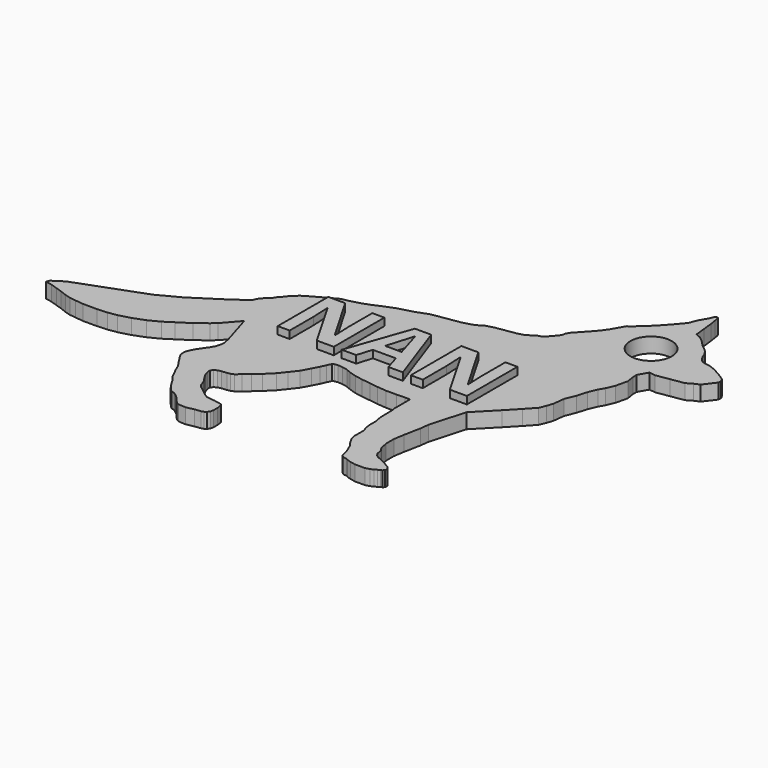
from build123d import *

# Parameters (mm, degrees)
F1_DEPTH     = 2
F2_TEXT_SIZE = 11.7813030051
F3_DEPTH     = 1
F4_R         = 2.75
F5_DEPTH     = 25


# Not quite as in the source:
# - Text() gives the source's letters only with a copy of the font that has no kerning and outlines rounded to 1/6400 em; it was checked with that copy


with BuildPart() as f1:
    # F0 (on Top) → F1 (new body)
    with BuildSketch(Plane.XY):
        Polygon((-14.7642782829, 2.6646352451), (-14.9479145184, 2.8952443972), (-15.7733522356, 3.3807961736), (-16.5259577334, 3.7813764066), (-17.0175787061, 3.969527781), (-17.4302980304, 4.218372982), (-17.7094899118, 4.7039249912), (-17.8126692772, 5.3533501923), (-18.1480534375, 5.8560813777), (-18.3847602457, 6.9182254374), (-18.3847602457, 8.2523440942), (-18.1536488235, 9.6542872488), (-17.7318826318, 11.7992078885), (-17.5875257701, 12.9829216748), (-16.272848472, 17.6499541849), (-13.6595489457, 20.3296020627), (-12.1902143583, 21.8657236546), (-11.032557115, 23.134695366), (-10.6763551012, 23.9806752652), (-10.4058505967, 24.8027704656), (-10.2194390335, 26.3313291684), (-9.6577452496, 27.7172196656), (-9.2633534223, 29.0438104421), (-8.7972544134, 30.1552768797), (-8.3670094609, 30.9082064778), (-7.900910452, 31.9838188589), (-7.5293937698, 33.5728228092), (-7.7079210069, 34.6964979394), (-7.7079210069, 35.2647826076), (-7.0022613507, 36.4996885333), (-6.1550052792, 36.3963635328), (-4.3928318448, 36.676334092), (-2.6384201724, 36.955071478), (-1.8559044693, 37.4121628702), (-1.1538827093, 37.7210527658), (0, 39.2280593514), (0, 39.6919772029), (-0.186430887, 40.0440022349), (-0.7630236214, 40.4506511986), (-1.4578301318, 40.8476829992), (-2.1245303449, 41.2286540783), (-2.869104268, 41.5249355137), (-3.3008807804, 41.639059782), (-3.839620389, 41.7309626937), (-4.1983937845, 41.8413393199), (-4.5092995279, 42.101085186), (-4.9067870714, 42.7150242031), (-5.1091215573, 43.2863943279), (-5.4541163373, 43.8192556956), (-5.84711181, 44.1954396665), (-6.3063995913, 44.533226639), (-6.6842092201, 44.9110381305), (-7.2530955076, 45.4910211265), (-7.8333392739, 45.9576323628), (-8.3694400653, 46.1709580073), (-8.5414147635, 46.2692291419), (-8.6991982535, 47.6955734193), (-8.8518235205, 49.0752879662), (-8.9826229554, 49.898557706), (-9.0659948644, 50.4233120359), (-9.1758315062, 50.5929601192), (-9.4891982153, 50.5929601192), (-9.7224124552, 50.0068780339), (-10.3918244695, 48.8354055599), (-10.823905442, 47.7495588401), (-11.8327699602, 46.5355329216), (-13.1241520867, 45.1289601624), (-14.3222687766, 44.0244451165), (-14.98264962, 43.4156558528), (-15.3725821915, 43.1631986287), (-15.7134736528, 42.5666378337), (-16.0001238116, 42.0649994351), (-16.2765689786, 41.5812197945), (-16.7349204421, 40.9167297184), (-17.23238267, 40.298666805), (-17.6576314861, 39.8354860096), (-18.3152012842, 39.119261318), (-19.0280626321, 38.3428130984), (-19.3103955608, 37.8487298621), (-19.3617039295, 37.4280056746), (-19.9972675541, 36.6383611881), (-20.6916112409, 35.8820823956), (-21.2846137583, 35.7196964324), (-21.9872504849, 35.2647826076), (-22.359482599, 35.023785335), (-23.2757088866, 34.7728887808), (-24.6350625074, 34.5569174207), (-25.9600134084, 34.3464118953), (-26.8741886643, 34.0960769893), (-27.3343137064, 33.7981744817), (-28.0513148755, 33.4564000368), (-29.3728645899, 33.0945109772), (-32.9943805465, 32.5191318304), (-34.4937965274, 31.9499187171), (-35.3291881792, 31.7211576679), (-36.5398315465, 31.3896388572), (-37.9009395838, 30.8641251177), (-38.9118529856, 30.4148308933), (-40.2074381709, 29.9338065088), (-41.4481340094, 29.5940582229), (-42.3404090351, 29.4522953674), (-44.2115776241, 28.4506026655), (-45.6762202084, 27.63691172), (-46.1677952958, 27.3186472532), (-46.9191087923, 26.6260293571), (-47.3907393699, 26.0400605087), (-47.8320423142, 25.5593935649), (-48.0084507771, 25.250678373), (-48.6776196227, 24.6337876608), (-49.1095043646, 24.0972003042), (-49.2985032646, 23.76645182), (-49.4094442508, 23.4876501286), (-50.3779351711, 22.7679461241), (-51.8682226539, 21.74083516), (-53.6844248452, 20.564956567), (-55.3585457164, 19.4810668415), (-58.2330115139, 17.9671943188), (-60.9993263118, 16.9401179921), (-63.1499052094, 16.1416518609), (-65.6253903512, 15.2225546605), (-67.1430172165, 14.6590907239), (-67.9922492424, 14.1092655092), (-68.5793457839, 13.7291568085), (-68.7404349446, 13.3243295934), (-67.9002553225, 13.1457727402), (-66.9656321406, 12.8442794085), (-66.1365240812, 12.580472976), (-65.310678236, 12.251851754), (-64.5235329866, 12.0227104053), (-63.6781375514, 11.9196123141), (-62.5939816236, 11.7992078885), (-60.725428164, 11.7992078885), (-59.436544776, 11.8753025308), (-58.2228863229, 12.0681261367), (-56.7238231287, 12.4786249349), (-55.146021906, 13.0644303845), (-53.7442006171, 13.7826036662), (-52.5471928994, 14.5575921325), (-51.0051218843, 15.555987743), (-49.5827570558, 16.6421439499), (-48.9357076585, 17.1993039548), (-47.1326112747, 19.274013117), (-46.1794324219, 16.123868525), (-45.8431750551, 15.0125772678), (-45.686647296, 14.148584567), (-45.7275994122, 13.5787213221), (-45.903544873, 12.9678025842), (-46.2326109409, 12.3907737434), (-46.6284863651, 11.8433907628), (-47.1506491303, 11.0767642036), (-47.590509057, 10.1432800293), (-47.6344972849, 9.6496576443), (-47.5416369736, 9.209795855), (-47.3294369876, 8.8092219085), (-46.8210428953, 8.0125341192), (-46.1794324219, 7.0639397018), (-45.8553694189, 6.2951319851), (-45.4332754016, 5.4509514011), (-45.1647564769, 4.8778424971), (-44.8632612824, 4.5160511509), (-44.5316210389, 4.0638111532), (-44.1999770701, 3.4909744281), (-43.7551513314, 2.8255861253), (-43.1412085891, 2.1683548111), (-42.7279807627, 2.0857087802), (-42.3066094518, 1.7986688763), (-41.7989268899, 1.3736330438), (-41.4407961071, 0.877757906), (-41.0157591105, 0.4960127408), (-40.7481454313, 0.3503986809), (-39.7392772138, 0.2968001063), (-38.7640046393, 0.5026923139), (-37.9602834582, 0.5998159759), (-37.6323738544, 0.6990357072), (-37.3525731266, 0.8711700211), (-37.1583513916, 1.1989175109), (-37.0761806397, 1.6097689551), (-37.0761806397, 2.2914088331), (-37.1716208756, 2.9547144659), (-37.3415648937, 3.1428658403), (-37.7419091156, 3.2229351359), (-38.354685096, 3.3454910225), (-38.9863699675, 3.3977804706), (-39.5057719214, 3.5016614466), (-39.9210564792, 3.761944361), (-40.4794402421, 4.2110797949), (-41.3083918393, 4.8364941031), (-41.6098870337, 5.1681362092), (-41.7290975182, 5.4509514011), (-41.8746797606, 5.93208368), (-42.3636175692, 6.6831391305), (-42.7555590868, 7.3388866149), (-42.9591825533, 8.011838349), (-42.9591825533, 8.3781415597), (-42.700894177, 8.6512649432), (-42.3549376428, 8.8636940345), (-41.8997332454, 8.9608039707), (-41.1956831813, 9.0214982629), (-40.810323857, 9.1028524238), (-40.4135754926, 9.2700873041), (-39.8361384869, 9.7619649023), (-39.0434265137, 10.4023432359), (-38.1937101483, 11.1670875922), (-37.154879421, 12.1954074129), (-36.3993123174, 13.1485881284), (-35.608869046, 14.148264192), (-35.004414618, 15.2758071199), (-34.5510728657, 16.123868525), (-34.2372208834, 16.8218184263), (-33.9466147125, 17.4262747169), (-33.7131110188, 17.5246997282), (-33.2918912172, 17.5897069275), (-32.6484814286, 17.5271835178), (-31.9469312857, 17.3868726987), (-31.3260174269, 17.1076620489), (-30.3495973349, 16.8111361563), (-29.3578095734, 16.6421439499), (-28.1621385366, 16.4792723954), (-27.0514376462, 16.3336079568), (-25.8467271924, 16.220998019), (-24.4026593864, 16.220998019), (-23.3007147908, 16.2543058395), (-22.651353851, 16.2543058395), (-22.651353851, 14.9536281824), (-22.651353851, 13.6544294655), (-22.5785799892, 13.3097134009), (-22.5393231958, 11.1658675596), (-22.4855616689, 10.8677390963), (-22.4113747609, 10.516329698), (-22.3459558564, 10.3001278724), (-22.3459558564, 8.9810490608), (-22.2775026826, 8.6567992809), (-22.185575291, 8.2213565559), (-22.0307393203, 7.8540233893), (-22.0307393203, 6.2540732324), (-21.9347831768, 5.7995470693), (-21.8293042029, 5.4509514011), (-21.6393717692, 5.1331802285), (-21.4076892976, 4.7455581189), (-21.1743861437, 4.3898373842), (-20.9956821054, 4.1598370299), (-20.7182520648, 3.5016614466), (-20.524304235, 3.0415392272), (-20.4106256453, 2.5030651774), (-20.2702097232, 2.0390069828), (-20.0385861099, 1.8236420583), (-19.8493698967, 1.7385558888), (-19.515639171, 1.7112329369), (-19.2272849381, 1.5597250313), (-18.6799019575, 1.393554965), (-17.9778139619, 1.2531365747), (-16.6467633098, 1.2531365747), (-16.0980569012, 1.4191655711), (-15.7317477784, 1.5735698933), (-15.4055255962, 1.7685535115), (-15.1684349403, 1.9470051629), (-14.9271438504, 1.9979447223), (-14.7469509393, 2.2005296778), (-14.7077152703, 2.3967069173), align=None)
    extrude(amount=F1_DEPTH)

    # F2 (on face) → F3 (join)
    with BuildSketch(Plane.XY.offset(2)):
        with Locations((-43.5519069433, 19.0434660763)):
            Text('NAN', F2_TEXT_SIZE, font='Open Sans', font_style=FontStyle.BOLD, text_align=(TextAlign.LEFT, TextAlign.BOTTOM))
    extrude(amount=F3_DEPTH)

    # F4 (on face) → F5 (cut)
    with BuildSketch(Plane.XY.offset(2)):
        with Locations((-10.2233579382, 40.8072024584)):
            Circle(F4_R)
    extrude(amount=-F5_DEPTH, mode=Mode.SUBTRACT)


solid = f1.part
